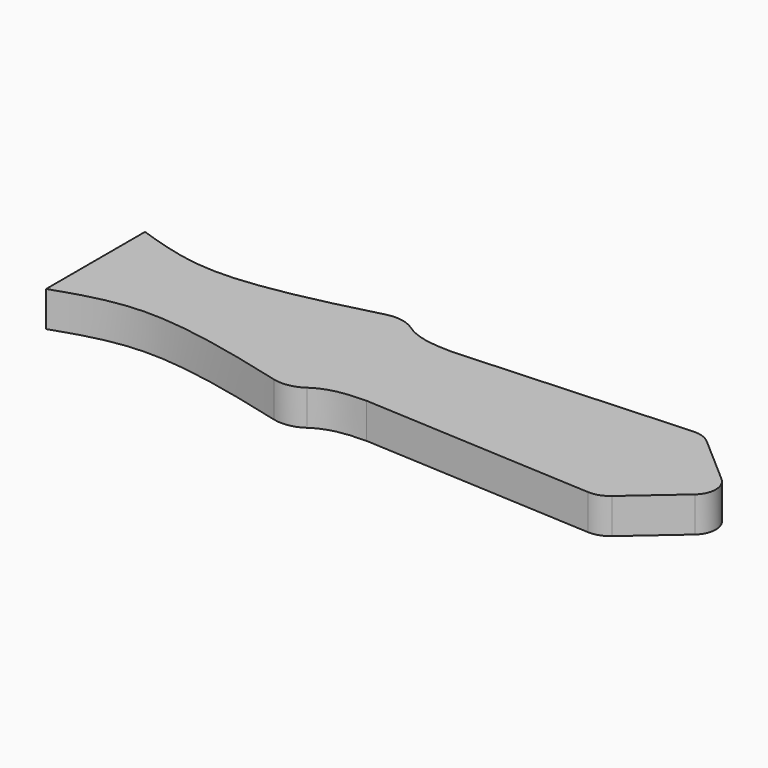
from build123d import *

# Parameters (mm, degrees)
F1_DEPTH = 4


with BuildPart() as f1:
    # F0 (on Top) → F1 (new body)
    with BuildSketch(Plane.XY):
        with BuildLine():
            Line((33.1839122816, 7.4341704185), (7, 6.0167759657))
            add(Edge.make_bspline(
                [(7, 6.0167759657), (4.0042999393, 6.0167759657), (2.4851097846, 6.5339730516), (1.3114110288, 7.3480597034)],
                knots=[0, 0, 0, 0, 5.2976431113, 5.2976431113, 5.2976431113, 5.2976431113], degree=3))
            ThreePointArc((1.3114110288, 7.3480597034), (-0.2690563082, 7.9996972089), (-1.9772483015, 7.9319583269))
            add(Edge.make_bspline(
                [(-1.9772483015, 7.9319583269), (-8.0874424423, 6.3392692714), (-18.8504021756, 3.7391038399), (-25.5343435285, 5.9978133829), (-28.5, 7)],
                knots=[0.0565322181, 0.0565322181, 0.0565322181, 0.0565322181, 0.5813845177, 1, 1, 1, 1], degree=3))
            Line((-28.5, 7), (-28.5, 0))
            Line((-28.5, 0), (-28.5, -7))
            add(Edge.make_bspline(
                [(-1.9772483015, -7.9319583269), (-8.0874424423, -6.3392692714), (-18.8504021756, -3.7391038399), (-25.5343435285, -5.9978133829), (-28.5, -7)],
                knots=[0.0565322181, 0.0565322181, 0.0565322181, 0.0565322181, 0.5813845177, 1, 1, 1, 1], degree=3))
            ThreePointArc((-1.9772483015, -7.9319583269), (-0.2690563082, -7.9996972089), (1.3114110288, -7.3480597034))
            add(Edge.make_bspline(
                [(7, -6.0167759657), (4.0042999393, -6.0167759657), (2.4851097846, -6.5339730516), (1.3114110288, -7.3480597034)],
                knots=[0, 0, 0, 0, 5.2976431113, 5.2976431113, 5.2976431113, 5.2976431113], degree=3))
            Line((7, -6.0167759657), (33.1839122816, -7.4341704185))
            ThreePointArc((33.1839122816, -7.4341704185), (34.3226011035, -7.2751722198), (35.3178602471, -6.6995404822))
            Line((35.3178602471, -6.6995404822), (40.8395039416, -1.8841535393))
            ThreePointArc((40.8395039416, -1.8841535393), (41.6963467853, 0), (40.8395039416, 1.8841535393))
            Line((40.8395039416, 1.8841535393), (35.3178602471, 6.6995404822))
            ThreePointArc((35.3178602471, 6.6995404822), (34.3226011035, 7.2751722198), (33.1839122816, 7.4341704185))
        make_face()
    extrude(amount=F1_DEPTH)


solid = f1.part
